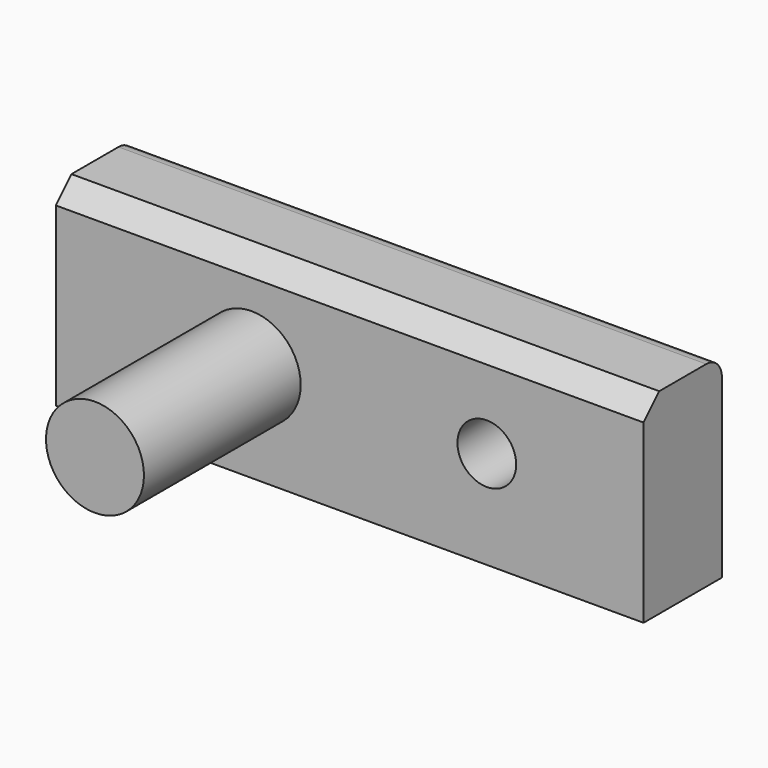
from build123d import *

# Parameters (mm, degrees)
F0_W     = 30
F0_H     = 10
F1_DEPTH = 5
F2_R     = 2.5
F3_DEPTH = 10
F4_R     = 1.5
F5_DEPTH = 5.001
F6_SIZE  = 1
F7_R     = 1


# Not quite as in the source:
# - a feature names something its author has since deleted; it is built from what else it names


with BuildPart() as f1:
    # F0 (on Front) → F1 (new body)
    with BuildSketch(Plane.XZ):
        with Locations((15, 10.7978725549)):
            Rectangle(F0_W, F0_H)
    extrude(amount=F1_DEPTH)

    # F2 (on face) → F3 (join)
    with BuildSketch(Plane.XZ.offset(5)):
        with Locations((10, 10.7978725549)):
            Circle(F2_R)
    extrude(amount=F3_DEPTH)

    # F4 (on face) → F5 (cut, through all)
    with BuildSketch(Plane.XZ.offset(5)):
        with Locations((22, 10.7978725549)):
            Circle(F4_R)
    extrude(amount=-F5_DEPTH, mode=Mode.SUBTRACT)

    # F6
    f6_edges = [f1.edges().sort_by_distance(p)[0] for p in [
        (15, -5, 15.797873),
    ]]
    chamfer(f6_edges, length=F6_SIZE)

    # F7
    f7_edges = [f1.edges().sort_by_distance(p)[0] for p in [
        (15, 0, 15.797873),
    ]]
    fillet(f7_edges, radius=F7_R)


solid = f1.part
